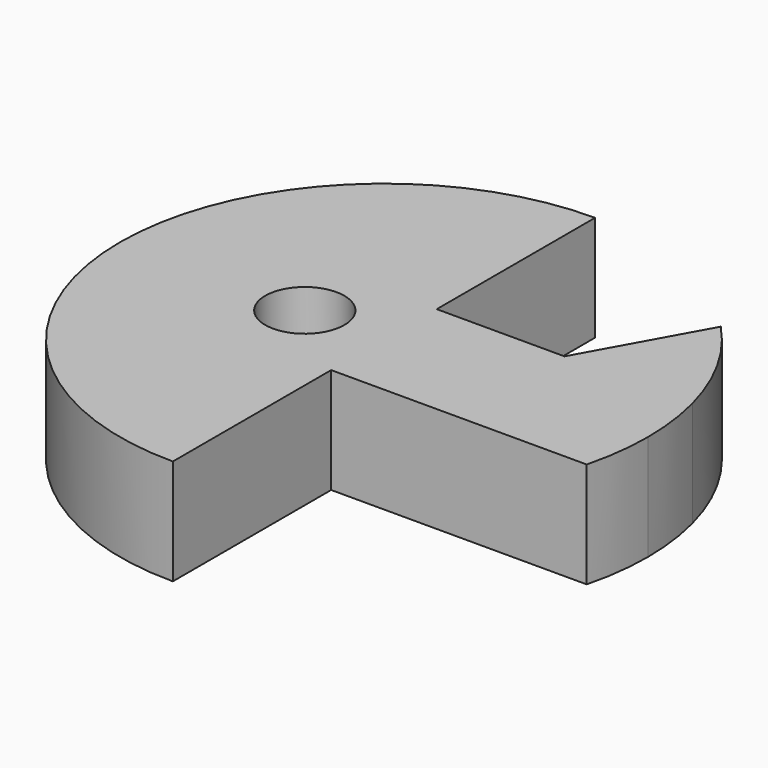
from build123d import *

# Parameters (mm, degrees)
F1_DEPTH = 5.08
F2_R     = 1.905
F3_DEPTH = 5.081


with BuildPart() as f1:
    # F0 (on Top) → F1 (new body)
    with BuildSketch(Plane.XY):
        with BuildLine():
            Line((0, 0), (12.7, 0))
            ThreePointArc((12.7, 0), (12.5987771426, 1.6002545145), (12.2967221242, 3.175))
            Line((12.2967221242, 3.175), (6.1483610621, 3.175))
            Line((6.1483610621, 3.175), (0, 3.175))
            Line((0, 3.175), (0, 0))
        make_face()
        with BuildLine():
            ThreePointArc((12.2967221242, -3.175), (12.5987771426, -1.6002545145), (12.7, 0))
            Line((12.7, 0), (0, 0))
            Line((0, 0), (0, -3.175))
            Line((0, -3.175), (6.1483610621, -3.175))
            Line((6.1483610621, -3.175), (12.2967221242, -3.175))
        make_face()
        with BuildLine():
            Line((6.1483610621, 3.175), (12.2967221242, 3.175))
            ThreePointArc((12.2967221242, 3.175), (11.1125, 6.1483610621), (9.2225415932, 8.73125))
            Line((9.2225415932, 8.73125), (6.1483610621, 3.175))
        make_face()
        with BuildLine():
            Line((-12.7, 0), (0, 0))
            Line((0, 0), (0, 3.175))
            Line((0, 3.175), (0, 6.35))
            Line((0, 6.35), (0, 12.7))
            ThreePointArc((0, 12.7), (-8.9802561211, 8.9802561211), (-12.7, 0))
        make_face()
        with BuildLine():
            Line((0, -3.175), (0, 0))
            Line((0, 0), (-12.7, 0))
            ThreePointArc((-12.7, 0), (-8.9802561211, -8.9802561211), (0, -12.7))
            Line((0, -12.7), (0, -6.35))
            Line((0, -6.35), (0, -3.175))
        make_face()
    extrude(amount=F1_DEPTH)

    # F2 (on face) → F3 (cut, through all)
    with BuildSketch(Plane.XY.offset(5.08)):
        with Locations((-3.81, 0)):
            Circle(F2_R)
    extrude(amount=-F3_DEPTH, mode=Mode.SUBTRACT)


solid = f1.part
